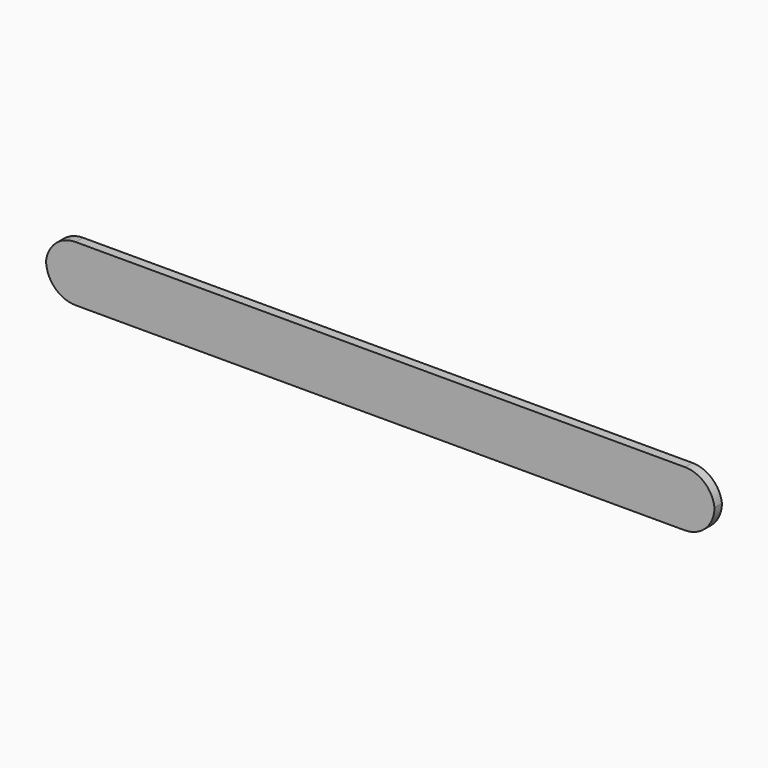
from build123d import *

# Parameters (mm, degrees)
F0_W        = 114.3
F0_H        = 9.525
F1_DEPTH    = 1.5875
F2_R        = 5.08
F3_T1_DEPTH = 26.7882812379
F4_R        = 5.08
F5_T1_DEPTH = 26.7882812379


# Not quite as in the source:
# - a fillet or chamfer that OpenCascade refuses, or shapes differently, is made with other operations: its cross-section is extruded or revolved along the edge and cut away or added


with BuildPart() as f1:
    # F0 (on Front) → F1 (new body)
    with BuildSketch(Plane.XZ):
        with Locations((-7.7723998189, 23.2028993189)):
            Rectangle(F0_W, F0_H)
    extrude(amount=F1_DEPTH)

    # F2
    f2_edges = [f1.edges().sort_by_distance(p)[0] for p in [
        (-64.9224, -0.79375, 18.440399),
    ]]
    fillet(f2_edges, radius=F2_R)

    # F3: fillet of radius 5.08 on 1 edges, made by hand

    # F3_s2 → F3_t1 (cut)
    with BuildSketch(Plane.XZ.offset(-12.6003906189)):
        with BuildLine():
            ThreePointArc((-64.9223998189, 23.5203993189), (-63.2423477364, 26.6953993189), (-59.8822435713, 27.9653993189))
            Line((-59.8822435713, 27.9653993189), (-64.9223998189, 27.9653993189))
            Line((-64.9223998189, 27.9653993189), (-64.9223998189, 23.5203993189))
        make_face()
    extrude(amount=F3_T1_DEPTH, mode=Mode.SUBTRACT)

    # F4
    f4_edges = [f1.edges().sort_by_distance(p)[0] for p in [
        (49.3776, -0.79375, 18.440399),
    ]]
    fillet(f4_edges, radius=F4_R)

    # F5: fillet of radius 5.08 on 1 edges, made by hand

    # F5_s2 → F5_t1 (cut)
    with BuildSketch(Plane.XZ.offset(-12.6003906189)):
        with BuildLine():
            ThreePointArc((49.3776001811, 23.5203993189), (47.6975480986, 26.6953993189), (44.3374439335, 27.9653993189))
            Line((44.3374439335, 27.9653993189), (49.3776001811, 27.9653993189))
            Line((49.3776001811, 27.9653993189), (49.3776001811, 23.5203993189))
        make_face()
    extrude(amount=F5_T1_DEPTH, mode=Mode.SUBTRACT)


solid = f1.part
